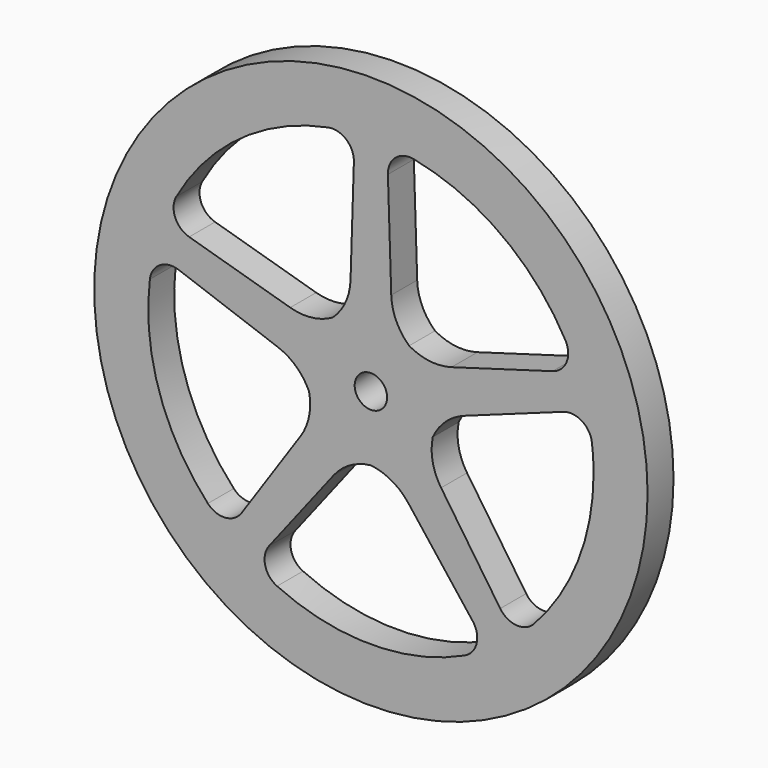
from build123d import *

# Parameters (mm, degrees)
F0_R        = 25.6
F0_R_2      = 1.5
F1_DEPTH    = 3
F2_COUNT    = 5
F3_T1_DEPTH = 3
F4_R        = 2


# Not quite as in the source:
# - a fillet or chamfer that OpenCascade refuses, or shapes differently, is made with other operations: its cross-section is extruded or revolved along the edge and cut away or added


with BuildPart() as f1:
    # F0 (on Front) → F1 (new body)
    with BuildSketch(Plane.XZ):
        Circle(F0_R)
        with BuildLine():
            ThreePointArc((-1.4990055262, 20.5453883495), (0, 20.6), (1.4990055262, 20.5453883495))
            ThreePointArc((1.4990055262, 20.5453883495), (15.0870725099, 14.0264123382), (20.6, 0))
            ThreePointArc((20.6, 0), (-14.0264123382, -15.0870725099), (-1.4990055262, 20.5453883495))
        make_face(mode=Mode.SUBTRACT)
        with BuildLine():
            ThreePointArc((-1.9720265944, 5.6666666667), (-3.4761933515, -4.8904069139), (6, 0))
            ThreePointArc((6, 0), (4.8904069139, 3.4761933515), (1.9720265944, 5.6666666667))
            ThreePointArc((1.9720265944, 5.6666666667), (0, 6), (-1.9720265944, 5.6666666667))
        make_face()
        Circle(F0_R_2, mode=Mode.SUBTRACT)
        with BuildLine():
            ThreePointArc((-1.9720265944, 5.6666666667), (0, 6), (1.9720265944, 5.6666666667))
            Line((1.9720265944, 5.6666666667), (1.4990055262, 20.5453883495))
            ThreePointArc((1.4990055262, 20.5453883495), (0, 20.6), (-1.4990055262, 20.5453883495))
            Line((-1.4990055262, 20.5453883495), (-1.9720265944, 5.6666666667))
        make_face()
    extrude(amount=F1_DEPTH)

    # F2: F1 ×5 about axis
    f2_axis = Axis((0, 0, 0), (0, -1, 0))


with BuildPart() as f1_1:
    add(f1.part)
    for i in range(1, F2_COUNT):
        add(f1.part.rotate(f2_axis, i * 360 / F2_COUNT))

    # F3: fillet of radius 5.08 on 10 edges, made by hand

    # F3_s2 → F3_t1 (join)
    with BuildSketch(Plane.XZ):
        with BuildLine():
            ThreePointArc((1.8832465894, 8.4592124416), (2.4124774845, 6.3578379743), (3.7693220099, 4.6682128899))
            ThreePointArc((3.7693220099, 4.6682128899), (2.9137601883, 5.244997766), (1.9720265944, 5.6666666667))
            Line((1.9720265944, 5.6666666667), (1.8832465894, 8.4592124416))
        make_face()
        with BuildLine():
            ThreePointArc((3.2749497301, 5.0273953759), (5.3011666938, 4.2590824136), (7.4632339146, 4.4051143441))
            Line((7.4632339146, 4.4051143441), (4.779930528, 3.6266050443))
            ThreePointArc((4.779930528, 3.6266050443), (4.0878878875, 4.3919440592), (3.2749497301, 5.0273953759))
        make_face()
        with BuildLine():
            ThreePointArc((5.7933522546, -1.5611116727), (5.6887786813, -3.7255802818), (6.4957788146, -5.7367020526))
            Line((6.4957788146, -5.7367020526), (4.9261861245, -3.4253014855))
            ThreePointArc((4.9261861245, -3.4253014855), (5.440213845, -2.5306270607), (5.7933522546, -1.5611116727))
        make_face()
        with BuildLine():
            ThreePointArc((-3.7693220099, 4.6682128899), (-2.4124774845, 6.3578379743), (-1.8832465894, 8.4592124416))
            Line((-1.8832465894, 8.4592124416), (-1.9720265944, 5.6666666667))
            ThreePointArc((-1.9720265944, 5.6666666667), (-2.9137601883, 5.244997766), (-3.7693220099, 4.6682128899))
        make_face()
        with BuildLine():
            ThreePointArc((-7.4632339146, 4.4051143441), (-5.3011666938, 4.2590824136), (-3.2749497301, 5.0273953759))
            ThreePointArc((-3.2749497301, 5.0273953759), (-4.0878878875, 4.3919440592), (-4.779930528, 3.6266050443))
            Line((-4.779930528, 3.6266050443), (-7.4632339146, 4.4051143441))
        make_face()
        with BuildLine():
            ThreePointArc((-5.6045188467, -2.1422811432), (-6.7921597763, -0.3297224505), (-8.627144316, 0.8229664629))
            Line((-8.627144316, 0.8229664629), (-5.99870999, -0.1244124414))
            ThreePointArc((-5.99870999, -0.1244124414), (-5.888690719, -1.1503571689), (-5.6045188467, -2.1422811432))
        make_face()
        with BuildLine():
            ThreePointArc((-6.4957788146, -5.7367020526), (-5.6887786813, -3.7255802818), (-5.7933522546, -1.5611116727))
            ThreePointArc((-5.7933522546, -1.5611116727), (-5.440213845, -2.5306270607), (-4.9261861245, -3.4253014855))
            Line((-4.9261861245, -3.4253014855), (-6.4957788146, -5.7367020526))
        make_face()
        with BuildLine():
            ThreePointArc((0.3055388721, -5.9922154499), (-1.7853081143, -6.5616176556), (-3.4486218238, -7.950591196))
            Line((-3.4486218238, -7.950591196), (-1.7353800681, -5.7435577841))
            ThreePointArc((-1.7353800681, -5.7435577841), (-0.7256508252, -5.9559575955), (0.3055388721, -5.9922154499))
        make_face()
        with BuildLine():
            ThreePointArc((3.4486218238, -7.950591196), (1.7853081143, -6.5616176556), (-0.3055388721, -5.9922154499))
            ThreePointArc((-0.3055388721, -5.9922154499), (0.7256508252, -5.9559575955), (1.7353800681, -5.7435577841))
            Line((1.7353800681, -5.7435577841), (3.4486218238, -7.950591196))
        make_face()
        with BuildLine():
            ThreePointArc((8.627144316, 0.8229664629), (6.7921597763, -0.3297224505), (5.6045188467, -2.1422811432))
            ThreePointArc((5.6045188467, -2.1422811432), (5.888690719, -1.1503571689), (5.99870999, -0.1244124414))
            Line((5.99870999, -0.1244124414), (8.627144316, 0.8229664629))
        make_face()
    extrude(amount=F3_T1_DEPTH)

    # F4
    f4_edges = [f1_1.edges().sort_by_distance(p)[0] for p in [
        (1.499006, -1.5, 20.545388),
        (-20.003044, -1.5, 4.923235),
        (20.003044, -1.5, 4.923235),
        (10.863555, -1.5, -17.502662),
        (-1.499006, -1.5, 20.545388),
        (19.076607, -1.5, 7.774513),
        (13.288997, -1.5, -15.740475),
        (-19.076607, -1.5, 7.774513),
        (-10.863555, -1.5, -17.502662),
        (-13.288997, -1.5, -15.740475),
    ]]
    fillet(f4_edges, radius=F4_R)


solid = f1_1.part
